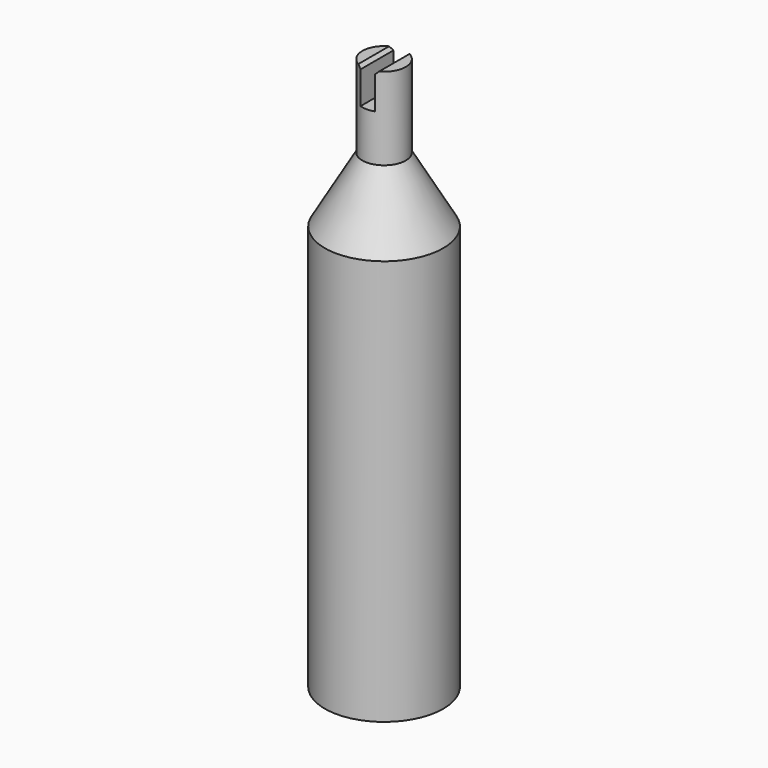
from build123d import *

# Parameters (mm, degrees)
F0_R        = 7.5
F0_R_2      = 2.75
F1_DEPTH    = 60
F2_DEPTH    = 10
F3_S5_R     = 2.75
F3_T6_DEPTH = 13
F5_DEPTH    = 4.5
F6_SIZE     = 0.4


# Not quite as in the source:
# - a fillet or chamfer that OpenCascade refuses, or shapes differently, is made with other operations: its cross-section is extruded or revolved along the edge and cut away or added


with BuildPart() as f1:
    # F0 (on Top) → F1 (new body)
    with BuildSketch(Plane.XY):
        Circle(F0_R)
        Circle(F0_R_2, mode=Mode.SUBTRACT)
        Circle(F0_R_2)
    extrude(amount=-F1_DEPTH)

    # F0 (on Top) → F2 (join)
    with BuildSketch(Plane.XY):
        Circle(F0_R_2)
    extrude(amount=F2_DEPTH)

    # F3: chamfer of 5 x 8.6602540378 on 1 edges, made by hand


with BuildPart() as f3_tool2:
    # F3_s3 → F3_t4 (revolve)
    with BuildSketch(Plane.XZ):
        Polygon((7.5, -8.6602540378), (2.5, 0), (7.5, 0), align=None)
    revolve(axis=Axis((0, 0, 0), (0, 0, 1)))

    # F3_s5 → F3_t6 (cut, symmetric)
    with BuildSketch(Plane.XY.offset(-4.3)):
        Circle(F3_S5_R)
    extrude(amount=F3_T6_DEPTH, both=True, mode=Mode.SUBTRACT)


with BuildPart() as f1_1:
    add(f1.part)

    # F3_t1: cut F3_tool2
    add(f3_tool2.part, mode=Mode.SUBTRACT)

    # F4 (on face) → F5 (cut)
    with BuildSketch(Plane.XY.offset(10)):
        with BuildLine():
            ThreePointArc((-0.9, -2.598557292), (0, -2.75), (0.9, -2.598557292))
            Line((0.9, -2.598557292), (0.9, 2.598557292))
            ThreePointArc((0.9, 2.598557292), (0, 2.75), (-0.9, 2.598557292))
            Line((-0.9, 2.598557292), (-0.9, -2.598557292))
        make_face()
        with BuildLine():
            ThreePointArc((-0.9, 2.598557292), (0, 2.75), (0.9, 2.598557292))
            Line((0.9, 2.598557292), (0.9, 4.5331302099))
            Line((0.9, 4.5331302099), (-0.9, 4.5331302099))
            Line((-0.9, 4.5331302099), (-0.9, 2.598557292))
        make_face()
    extrude(amount=-F5_DEPTH, mode=Mode.SUBTRACT)

    # F6
    f6_edges = [f1_1.edges().sort_by_distance(p)[0] for p in [
        (-0.9, 0, 10),
        (0.9, 0, 10),
    ]]
    chamfer(f6_edges, length=F6_SIZE)


solid = f1_1.part
